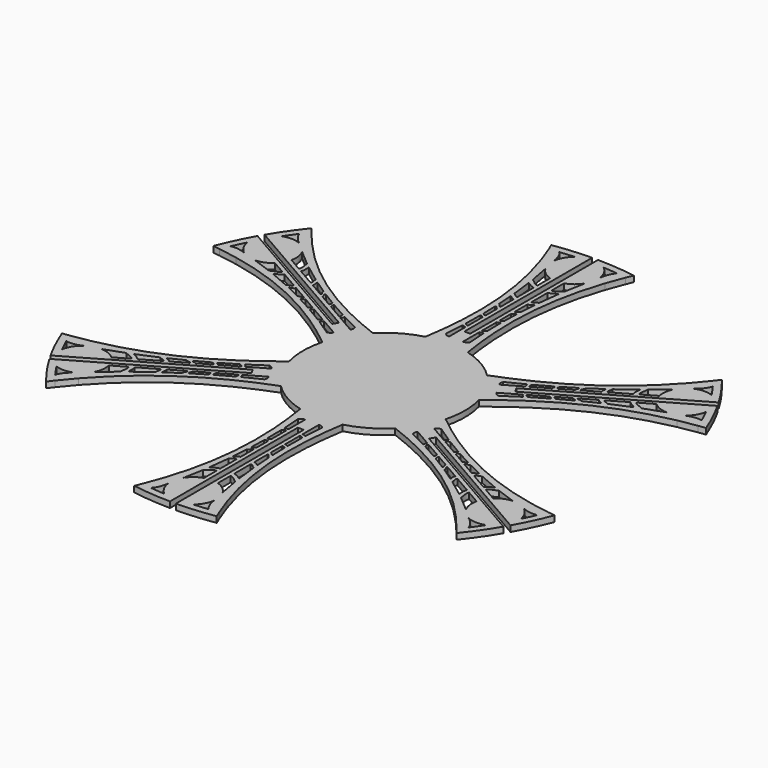
from build123d import *

# Parameters (mm, degrees)
F1_DEPTH = 6.35
F2_COUNT = 6


# Not quite as in the source:
# - a length typed as a fraction of an inch, garbled in the dataset ("3 / 203.2 mm" for 3/8 in), is restored


with BuildPart() as f1:
    # F0 (on Top) → F1 (new body)
    with BuildSketch(Plane.XY):
        with BuildLine():
            ThreePointArc((24.0985074366, 256.3698733068), (24.5345524636, 256.3285113588), (24.9705265041, 256.286407767))
            ThreePointArc((24.9705265041, 256.286407767), (24.9926305398, 256.8930249604), (25, 257.5))
            ThreePointArc((25, 257.5), (24.9791738801, 258.520231477), (24.9167302187, 259.5387631569))
            add(Edge.make_bspline(
                [(24.9167302187, 259.5387631569), (24.6398586668, 258.4897435126), (24.3671164775, 257.4333537767), (24.0985074366, 256.3698733068)],
                knots=[0, 0, 0, 0, 3.5683664228, 3.5683664228, 3.5683664228, 3.5683664228], degree=3))
        make_face()
        with BuildLine():
            ThreePointArc((3.175, 257.4804252269), (8.58681044, 257.3567886932), (13.9948260776, 257.1194174757))
            ThreePointArc((13.9948260776, 257.1194174757), (13.9987064596, 257.3096911541), (14, 257.5))
            ThreePointArc((14, 257.5), (10.9647161386, 266.2048836868), (3.175, 271.1352255207))
            Line((3.175, 271.1352255207), (3.175, 257.4804252269))
        make_face()
        with BuildLine():
            ThreePointArc((3.175, 243.8647744793), (10.845373305, 248.6468718593), (13.9948260776, 257.1194174757))
            ThreePointArc((13.9948260776, 257.1194174757), (8.58681044, 257.3567886932), (3.175, 257.4804252269))
            Line((3.175, 257.4804252269), (3.175, 243.8647744793))
        make_face()
        with BuildLine():
            add(Edge.make_bspline(
                [(34.4843217984, 255.1804881846), (12.7673180552, 190.6958065236), (15.0100402945, 133.2556042085), (22.8586233116, 84.4614310813)],
                knots=[23.4362562465, 23.4362562465, 23.4362562465, 23.4362562465, 198.2251842843, 198.2251842843, 198.2251842843, 198.2251842843], degree=3))
            ThreePointArc((34.4843217984, 255.1804881846), (29.7325665088, 255.7776856741), (24.9705265041, 256.286407767))
            ThreePointArc((24.9705265041, 256.286407767), (23.8907786453, 250.1358506449), (21.3204293609, 244.4447599844))
            add(Edge.make_bspline(
                [(21.3204293609, 244.4447599844), (19.7994681494, 237.3520104746), (18.447355185, 230.0121057952), (17.2650740181, 222.4976243712)],
                knots=[16.6038056007, 16.6038056007, 16.6038056007, 16.6038056007, 39.3732202874, 39.3732202874, 39.3732202874, 39.3732202874], degree=3))
            add(Edge.make_bspline(
                [(17.2650740181, 222.4976243712), (16.9207728297, 220.3092744624), (16.5908746927, 218.106119094), (16.2754038982, 215.8899507729)],
                knots=[39.3732202874, 39.3732202874, 39.3732202874, 39.3732202874, 46.0040765958, 46.0040765958, 46.0040765958, 46.0040765958], degree=3))
            add(Edge.make_bspline(
                [(16.2754038982, 215.8899507729), (15.1982070664, 208.3226908689), (14.2892226929, 200.6037092753), (13.5494178472, 192.8043682385)],
                knots=[46.0040765958, 46.0040765958, 46.0040765958, 46.0040765958, 68.6455937548, 68.6455937548, 68.6455937548, 68.6455937548], degree=3))
            add(Edge.make_bspline(
                [(13.5494178472, 192.8043682385), (13.377969648, 190.9968875439), (13.2156075865, 189.1850909786), (13.0623436996, 187.3698667527)],
                knots=[68.6455937548, 68.6455937548, 68.6455937548, 68.6455937548, 73.8927171936, 73.8927171936, 73.8927171936, 73.8927171936], degree=3))
            add(Edge.make_bspline(
                [(13.0623436996, 187.3698667527), (12.5830867073, 181.6936509129), (12.1927931423, 175.9839188521), (11.891831041, 170.2678288119)],
                knots=[73.8927171936, 73.8927171936, 73.8927171936, 73.8927171936, 90.3005001836, 90.3005001836, 90.3005001836, 90.3005001836], degree=3))
            add(Edge.make_bspline(
                [(11.891831041, 170.2678288119), (11.7934037382, 168.3984262432), (11.7045310241, 166.5283436467), (11.6252257724, 164.6585309992)],
                knots=[90.3005001836, 90.3005001836, 90.3005001836, 90.3005001836, 95.6665373615, 95.6665373615, 95.6665373615, 95.6665373615], degree=3))
            add(Edge.make_bspline(
                [(11.6252257724, 164.6585309992), (11.3941013481, 159.2092150662), (11.244238371, 153.7621919503), (11.1759555056, 148.3409766337)],
                knots=[95.6665373615, 95.6665373615, 95.6665373615, 95.6665373615, 111.3051265697, 111.3051265697, 111.3051265697, 111.3051265697], degree=3))
            add(Edge.make_bspline(
                [(11.1759555056, 148.3409766337), (11.1574760355, 146.8738269174), (11.1449715921, 145.4085673957), (11.1384484917, 143.9456641674)],
                knots=[111.3051265697, 111.3051265697, 111.3051265697, 111.3051265697, 115.5374158962, 115.5374158962, 115.5374158962, 115.5374158962], degree=3))
            add(Edge.make_bspline(
                [(11.1384484917, 143.9456641674), (11.1095814634, 137.471799521), (11.1978516102, 131.0440799553), (11.40380634, 124.7028999515)],
                knots=[115.5374158962, 115.5374158962, 115.5374158962, 115.5374158962, 134.2667943778, 134.2667943778, 134.2667943778, 134.2667943778], degree=3))
            add(Edge.make_bspline(
                [(11.40380634, 124.7028999515), (11.449861348, 123.2849034052), (11.5018011295, 121.8712342374), (11.5596318056, 120.4623441347)],
                knots=[134.2667943778, 134.2667943778, 134.2667943778, 134.2667943778, 138.4550044562, 138.4550044562, 138.4550044562, 138.4550044562], degree=3))
            add(Edge.make_bspline(
                [(11.5596318056, 120.4623441347), (11.848732793, 113.4191700443), (12.2850527804, 106.495429289), (12.869356484, 99.7475520216)],
                knots=[138.4550044562, 138.4550044562, 138.4550044562, 138.4550044562, 159.3922604228, 159.3922604228, 159.3922604228, 159.3922604228], degree=3))
            add(Edge.make_bspline(
                [(12.869356484, 99.7475520216), (13.2640628297, 95.1892547518), (13.7262973279, 90.7112077739), (14.2562957042, 86.3308058157)],
                knots=[159.3922604228, 159.3922604228, 159.3922604228, 159.3922604228, 173.5357062692, 173.5357062692, 173.5357062692, 173.5357062692], degree=3))
            ThreePointArc((14.2562957042, 86.3308058157), (18.5809833933, 85.5043686377), (22.8586233116, 84.4614310813))
        make_face()
        with BuildLine():
            ThreePointArc((24.9705265041, 256.286407767), (29.7325665088, 255.7776856741), (34.4843217984, 255.1804881846))
            add(Edge.make_bspline(
                [(41.5870895219, 274.3661130408), (38.9772182382, 267.9040789576), (36.6154101026, 261.5083662156), (34.4843217984, 255.1804881846)],
                knots=[6.284228985, 6.284228985, 6.284228985, 6.284228985, 23.4362562465, 23.4362562465, 23.4362562465, 23.4362562465], degree=3))
            ThreePointArc((41.5870895219, 274.3661130408), (36.492945437, 275.0900124202), (31.3862552738, 275.719337334))
            add(Edge.make_bspline(
                [(31.3862552738, 275.719337334), (28.0236396939, 273.0873525143), (25.1960325986, 265.6025290489), (24.8841398376, 259.9040766508)],
                knots=[0, 0, 0, 0, 17.0997068871, 17.0997068871, 17.0997068871, 17.0997068871], degree=3))
            ThreePointArc((24.8841398376, 259.9040766508), (24.901104957, 259.7214796696), (24.9167302187, 259.5387631569))
            ThreePointArc((24.9167302187, 259.5387631569), (24.9791738801, 258.520231477), (25, 257.5))
            ThreePointArc((25, 257.5), (24.9926305398, 256.8930249604), (24.9705265041, 256.286407767))
        make_face()
        with BuildLine():
            ThreePointArc((87.5, 0), (69.4851766198, 53.1795094949), (22.8586233116, 84.4614310813))
            ThreePointArc((22.8586233116, 84.4614310813), (18.5809833933, 85.5043686377), (14.2562957042, 86.3308058157))
            ThreePointArc((14.2562957042, 86.3308058157), (10.8863917915, 86.8201386417), (7.5, 87.1779788708))
            ThreePointArc((7.5, 87.1779788708), (5.3391369062, 87.3369544757), (3.175, 87.4423774551))
            ThreePointArc((3.175, 87.4423774551), (0, 87.5), (-3.175, 87.4423774551))
            ThreePointArc((-3.175, 87.4423774551), (-5.3391369062, 87.3369544757), (-7.5, 87.1779788708))
            ThreePointArc((-7.5, 87.1779788708), (-10.8863917915, 86.8201386417), (-14.2562957042, 86.3308058157))
            ThreePointArc((-14.2562957042, 86.3308058157), (-18.5809833933, 85.5043686377), (-22.8586233116, 84.4614310813))
            ThreePointArc((-22.8586233116, 84.4614310813), (-53.1795094949, -69.4851766198), (87.5, 0))
        make_face()
        with BuildLine():
            add(Edge.make_bspline(
                [(-41.5870895219, 274.3661130408), (-38.9772182382, 267.9040789576), (-36.6154101026, 261.5083662156), (-34.4843217984, 255.1804881846)],
                knots=[6.284228985, 6.284228985, 6.284228985, 6.284228985, 23.4362562465, 23.4362562465, 23.4362562465, 23.4362562465], degree=3))
            ThreePointArc((-34.4843217984, 255.1804881846), (-29.7325665088, 255.7776856741), (-24.9705265041, 256.286407767))
            ThreePointArc((-24.9705265041, 256.286407767), (-24.9965807607, 257.9134613325), (-24.9167302187, 259.5387631569))
            ThreePointArc((-24.9167302187, 259.5387631569), (-24.901104957, 259.7214796696), (-24.8841398376, 259.9040766508))
            add(Edge.make_bspline(
                [(-31.3862552738, 275.719337334), (-28.0236396939, 273.0873525143), (-25.1960325986, 265.6025290489), (-24.8841398376, 259.9040766508)],
                knots=[0, 0, 0, 0, 17.0997068871, 17.0997068871, 17.0997068871, 17.0997068871], degree=3))
            ThreePointArc((-31.3862552738, 275.719337334), (-36.492945437, 275.0900124202), (-41.5870895219, 274.3661130408))
        make_face()
        with BuildLine():
            ThreePointArc((-24.9705265041, 256.286407767), (-29.7325665088, 255.7776856741), (-34.4843217984, 255.1804881846))
            add(Edge.make_bspline(
                [(-34.4843217984, 255.1804881846), (-12.7673180552, 190.6958065236), (-15.0100402945, 133.2556042085), (-22.8586233116, 84.4614310813)],
                knots=[23.4362562465, 23.4362562465, 23.4362562465, 23.4362562465, 198.2251842843, 198.2251842843, 198.2251842843, 198.2251842843], degree=3))
            ThreePointArc((-22.8586233116, 84.4614310813), (-18.5809833933, 85.5043686377), (-14.2562957042, 86.3308058157))
            add(Edge.make_bspline(
                [(-12.869356484, 99.7475520216), (-13.2640628297, 95.1892547518), (-13.7262973279, 90.7112077739), (-14.2562957042, 86.3308058157)],
                knots=[159.3922604228, 159.3922604228, 159.3922604228, 159.3922604228, 173.5357062692, 173.5357062692, 173.5357062692, 173.5357062692], degree=3))
            add(Edge.make_bspline(
                [(-11.5596318056, 120.4623441347), (-11.848732793, 113.4191700443), (-12.2850527804, 106.495429289), (-12.869356484, 99.7475520216)],
                knots=[138.4550044562, 138.4550044562, 138.4550044562, 138.4550044562, 159.3922604228, 159.3922604228, 159.3922604228, 159.3922604228], degree=3))
            add(Edge.make_bspline(
                [(-11.40380634, 124.7028999515), (-11.449861348, 123.2849034052), (-11.5018011295, 121.8712342374), (-11.5596318056, 120.4623441347)],
                knots=[134.2667943778, 134.2667943778, 134.2667943778, 134.2667943778, 138.4550044562, 138.4550044562, 138.4550044562, 138.4550044562], degree=3))
            add(Edge.make_bspline(
                [(-11.1384484917, 143.9456641674), (-11.1095814634, 137.471799521), (-11.1978516102, 131.0440799553), (-11.40380634, 124.7028999515)],
                knots=[115.5374158962, 115.5374158962, 115.5374158962, 115.5374158962, 134.2667943778, 134.2667943778, 134.2667943778, 134.2667943778], degree=3))
            add(Edge.make_bspline(
                [(-11.1759555056, 148.3409766337), (-11.1574760355, 146.8738269174), (-11.1449715921, 145.4085673957), (-11.1384484917, 143.9456641674)],
                knots=[111.3051265697, 111.3051265697, 111.3051265697, 111.3051265697, 115.5374158962, 115.5374158962, 115.5374158962, 115.5374158962], degree=3))
            add(Edge.make_bspline(
                [(-11.6252257724, 164.6585309992), (-11.3941013481, 159.2092150662), (-11.244238371, 153.7621919503), (-11.1759555056, 148.3409766337)],
                knots=[95.6665373615, 95.6665373615, 95.6665373615, 95.6665373615, 111.3051265697, 111.3051265697, 111.3051265697, 111.3051265697], degree=3))
            add(Edge.make_bspline(
                [(-11.891831041, 170.2678288119), (-11.7934037382, 168.3984262432), (-11.7045310241, 166.5283436467), (-11.6252257724, 164.6585309992)],
                knots=[90.3005001836, 90.3005001836, 90.3005001836, 90.3005001836, 95.6665373615, 95.6665373615, 95.6665373615, 95.6665373615], degree=3))
            add(Edge.make_bspline(
                [(-13.0623436996, 187.3698667527), (-12.5830867073, 181.6936509129), (-12.1927931423, 175.9839188521), (-11.891831041, 170.2678288119)],
                knots=[73.8927171936, 73.8927171936, 73.8927171936, 73.8927171936, 90.3005001836, 90.3005001836, 90.3005001836, 90.3005001836], degree=3))
            add(Edge.make_bspline(
                [(-13.5494178472, 192.8043682385), (-13.377969648, 190.9968875439), (-13.2156075865, 189.1850909786), (-13.0623436996, 187.3698667527)],
                knots=[68.6455937548, 68.6455937548, 68.6455937548, 68.6455937548, 73.8927171936, 73.8927171936, 73.8927171936, 73.8927171936], degree=3))
            add(Edge.make_bspline(
                [(-16.2754038982, 215.8899507729), (-15.1982070664, 208.3226908689), (-14.2892226929, 200.6037092753), (-13.5494178472, 192.8043682385)],
                knots=[46.0040765958, 46.0040765958, 46.0040765958, 46.0040765958, 68.6455937548, 68.6455937548, 68.6455937548, 68.6455937548], degree=3))
            add(Edge.make_bspline(
                [(-17.2650740181, 222.4976243712), (-16.9207728297, 220.3092744624), (-16.5908746927, 218.106119094), (-16.2754038982, 215.8899507729)],
                knots=[39.3732202874, 39.3732202874, 39.3732202874, 39.3732202874, 46.0040765958, 46.0040765958, 46.0040765958, 46.0040765958], degree=3))
            add(Edge.make_bspline(
                [(-21.3204293609, 244.4447599844), (-19.7994681494, 237.3520104746), (-18.447355185, 230.0121057952), (-17.2650740181, 222.4976243712)],
                knots=[16.6038056007, 16.6038056007, 16.6038056007, 16.6038056007, 39.3732202874, 39.3732202874, 39.3732202874, 39.3732202874], degree=3))
            ThreePointArc((-21.3204293609, 244.4447599844), (-23.8907786453, 250.1358506449), (-24.9705265041, 256.286407767))
        make_face()
        with BuildLine():
            add(Edge.make_bspline(
                [(-17.2650740181, 222.4976243712), (-13.0134568191, 219.9089487239), (-11.2873415643, 216.6422307491), (-7.5, 216.5923267603)],
                knots=[0, 0, 0, 0, 11.4118013675, 11.4118013675, 11.4118013675, 11.4118013675], degree=3))
            add(Edge.make_bspline(
                [(-17.2650740181, 222.4976243712), (-16.9207728297, 220.3092744624), (-16.5908746927, 218.106119094), (-16.2754038982, 215.8899507729)],
                knots=[39.3732202874, 39.3732202874, 39.3732202874, 39.3732202874, 46.0040765958, 46.0040765958, 46.0040765958, 46.0040765958], degree=3))
            add(Edge.make_bspline(
                [(-16.2754038982, 215.8899507729), (-12.5103608703, 213.8302643566), (-11.8700430909, 212.4467641115), (-7.5, 211.5250229836)],
                knots=[0, 0, 0, 0, 9.801036077, 9.801036077, 9.801036077, 9.801036077], degree=3))
            Line((-7.5, 211.5250229836), (-7.5, 216.5923267603))
        make_face()
        with BuildLine():
            add(Edge.make_bspline(
                [(-13.5494178472, 192.8043682385), (-10.0457689154, 191.3002797398), (-10.2384781645, 189.022153616), (-7.5, 189.5666867495)],
                knots=[0, 0, 0, 0, 6.8613437252, 6.8613437252, 6.8613437252, 6.8613437252], degree=3))
            add(Edge.make_bspline(
                [(-13.5494178472, 192.8043682385), (-13.377969648, 190.9968875439), (-13.2156075865, 189.1850909786), (-13.0623436996, 187.3698667527)],
                knots=[68.6455937548, 68.6455937548, 68.6455937548, 68.6455937548, 73.8927171936, 73.8927171936, 73.8927171936, 73.8927171936], degree=3))
            add(Edge.make_bspline(
                [(-13.0623436996, 187.3698667527), (-10.2409727406, 186.262742786), (-10.2384781645, 184.243991971), (-7.5, 184.4993829727)],
                knots=[0, 0, 0, 0, 6.2593405854, 6.2593405854, 6.2593405854, 6.2593405854], degree=3))
            Line((-7.5, 184.4993829727), (-7.5, 189.5666867495))
        make_face()
        with BuildLine():
            add(Edge.make_bspline(
                [(-11.891831041, 170.2678288119), (-9.259641322, 169.3483605489), (-9.8297276348, 166.1768704653), (-7.5, 166.491702199)],
                knots=[0, 0, 0, 0, 5.7920041513, 5.7920041513, 5.7920041513, 5.7920041513], degree=3))
            add(Edge.make_bspline(
                [(-11.891831041, 170.2678288119), (-11.7934037382, 168.3984262432), (-11.7045310241, 166.5283436467), (-11.6252257724, 164.6585309992)],
                knots=[90.3005001836, 90.3005001836, 90.3005001836, 90.3005001836, 95.6665373615, 95.6665373615, 95.6665373615, 95.6665373615], degree=3))
            add(Edge.make_bspline(
                [(-11.6252257724, 164.6585309992), (-8.90752234, 165.1033413686), (-9.8926938884, 162.4619066715), (-7.5, 162.2730046511)],
                knots=[0, 0, 0, 0, 4.7653146413, 4.7653146413, 4.7653146413, 4.7653146413], degree=3))
            Line((-7.5, 162.2730046511), (-7.5, 166.491702199))
        make_face()
        with BuildLine():
            add(Edge.make_bspline(
                [(-11.1759555056, 148.3409766337), (-11.1574760355, 146.8738269174), (-11.1449715921, 145.4085673957), (-11.1384484917, 143.9456641674)],
                knots=[111.3051265697, 111.3051265697, 111.3051265697, 111.3051265697, 115.5374158962, 115.5374158962, 115.5374158962, 115.5374158962], degree=3))
            add(Edge.make_bspline(
                [(-11.1384484917, 143.9456641674), (-8.4912590683, 144.0353989601), (-9.1877372184, 142.4406170845), (-7.5, 142.7544057369)],
                knots=[0, 0, 0, 0, 3.8284989323, 3.8284989323, 3.8284989323, 3.8284989323], degree=3))
            Line((-7.5, 142.7544057369), (-7.5, 146.8565165997))
            add(Edge.make_bspline(
                [(-11.1759555056, 148.3409766337), (-9.7026852891, 146.906927228), (-9.2796140531, 146.3913172483), (-7.5, 146.8565165997)],
                knots=[0, 0, 0, 0, 3.9643751679, 3.9643751679, 3.9643751679, 3.9643751679], degree=3))
        make_face()
        with BuildLine():
            add(Edge.make_bspline(
                [(-11.40380634, 124.7028999515), (-11.449861348, 123.2849034052), (-11.5018011295, 121.8712342374), (-11.5596318056, 120.4623441347)],
                knots=[134.2667943778, 134.2667943778, 134.2667943778, 134.2667943778, 138.4550044562, 138.4550044562, 138.4550044562, 138.4550044562], degree=3))
            add(Edge.make_bspline(
                [(-11.5596318056, 120.4623441347), (-9.5880907525, 119.8675970578), (-9.5183962158, 119.5819102936), (-7.5, 119.7053417563)],
                knots=[0, 0, 0, 0, 4.1296080926, 4.1296080926, 4.1296080926, 4.1296080926], degree=3))
            Line((-7.5, 119.7053417563), (-7.5, 122.7562793089))
            add(Edge.make_bspline(
                [(-11.40380634, 124.7028999515), (-9.5969793375, 123.429948461), (-9.4491818808, 122.6324219398), (-7.5, 122.7562793089)],
                knots=[0, 0, 0, 0, 4.3622283143, 4.3622283143, 4.3622283143, 4.3622283143], degree=3))
        make_face()
        with BuildLine():
            add(Edge.make_bspline(
                [(-12.869356484, 99.7475520216), (-13.2640628297, 95.1892547518), (-13.7262973279, 90.7112077739), (-14.2562957042, 86.3308058157)],
                knots=[159.3922604228, 159.3922604228, 159.3922604228, 159.3922604228, 173.5357062692, 173.5357062692, 173.5357062692, 173.5357062692], degree=3))
            ThreePointArc((-14.2562957042, 86.3308058157), (-10.8863917915, 86.8201386417), (-7.5, 87.1779788708))
            Line((-7.5, 87.1779788708), (-7.5, 97.2476452589))
            add(Edge.make_bspline(
                [(-12.869356484, 99.7475520216), (-10.8381348679, 97.5883237043), (-10.0787932936, 97.1908478477), (-7.5, 97.2476452589)],
                knots=[0, 0, 0, 0, 5.9227968794, 5.9227968794, 5.9227968794, 5.9227968794], degree=3))
        make_face()
        with BuildLine():
            ThreePointArc((21.3204293609, 244.4447599844), (23.8907786453, 250.1358506449), (24.9705265041, 256.286407767))
            ThreePointArc((24.9705265041, 256.286407767), (24.5345524636, 256.3285113588), (24.0985074366, 256.3698733068))
            add(Edge.make_bspline(
                [(24.0985074366, 256.3698733068), (23.1172638083, 252.4849205467), (22.1911762658, 248.5053432761), (21.3204293609, 244.4447599844)],
                knots=[3.5683664228, 3.5683664228, 3.5683664228, 3.5683664228, 16.6038056007, 16.6038056007, 16.6038056007, 16.6038056007], degree=3))
        make_face()
        with BuildLine():
            ThreePointArc((-24.0985074366, 256.3698733068), (-24.5345524636, 256.3285113588), (-24.9705265041, 256.286407767))
            ThreePointArc((-24.9705265041, 256.286407767), (-23.8907786453, 250.1358506449), (-21.3204293609, 244.4447599844))
            add(Edge.make_bspline(
                [(-24.0985074366, 256.3698733068), (-23.1172638083, 252.4849205467), (-22.1911762658, 248.5053432761), (-21.3204293609, 244.4447599844)],
                knots=[3.5683664228, 3.5683664228, 3.5683664228, 3.5683664228, 16.6038056007, 16.6038056007, 16.6038056007, 16.6038056007], degree=3))
        make_face()
        with BuildLine():
            ThreePointArc((-24.9167302187, 259.5387631569), (-24.9965807607, 257.9134613325), (-24.9705265041, 256.286407767))
            ThreePointArc((-24.9705265041, 256.286407767), (-24.5345524636, 256.3285113588), (-24.0985074366, 256.3698733068))
            add(Edge.make_bspline(
                [(-24.9167302187, 259.5387631569), (-24.6398586668, 258.4897435126), (-24.3671164775, 257.4333537767), (-24.0985074366, 256.3698733068)],
                knots=[0, 0, 0, 0, 3.5683664228, 3.5683664228, 3.5683664228, 3.5683664228], degree=3))
        make_face()
        with BuildLine():
            add(Edge.make_bspline(
                [(24.0985074366, 256.3698733068), (23.1172638083, 252.4849205467), (22.1911762658, 248.5053432761), (21.3204293609, 244.4447599844)],
                knots=[3.5683664228, 3.5683664228, 3.5683664228, 3.5683664228, 16.6038056007, 16.6038056007, 16.6038056007, 16.6038056007], degree=3))
            ThreePointArc((24.0985074366, 256.3698733068), (19.0503535051, 256.794341899), (13.9948260776, 257.1194174757))
            ThreePointArc((13.9948260776, 257.1194174757), (10.845373305, 248.6468718593), (3.175, 243.8647744793))
            Line((3.175, 243.8647744793), (3.175, 232.7024320749))
            ThreePointArc((3.175, 232.7024320749), (5.358553742, 233.0810339737), (7.5, 233.6515199646))
            ThreePointArc((7.5, 233.6515199646), (15.3875857323, 237.7966448204), (21.3204293609, 244.4447599844))
        make_face()
        with BuildLine():
            ThreePointArc((31.3862552738, 275.719337334), (36.492945437, 275.0900124202), (41.5870895219, 274.3661130408))
            add(Edge.make_bspline(
                [(44.5564859897, 281.4955053926), (43.532819192, 279.1101881008), (42.543304698, 276.7336991732), (41.5870895219, 274.3661130408)],
                knots=[0, 0, 0, 0, 6.284228985, 6.284228985, 6.284228985, 6.284228985], degree=3))
            ThreePointArc((44.5564859897, 281.4955053926), (23.9293365456, 283.9936387536), (3.175, 284.9823141442))
            Line((3.175, 284.9823141442), (3.175, 282.2975679251))
            ThreePointArc((3.175, 282.2975679251), (9.7289002268, 280.5292965672), (15.5655019991, 277.0631067961))
            ThreePointArc((15.5655019991, 277.0631067961), (23.4854914116, 276.5043972402), (31.3862552738, 275.719337334))
        make_face()
        with BuildLine():
            ThreePointArc((13.9948260776, 257.1194174757), (19.0503535051, 256.794341899), (24.0985074366, 256.3698733068))
            add(Edge.make_bspline(
                [(24.9167302187, 259.5387631569), (24.6398586668, 258.4897435126), (24.3671164775, 257.4333537767), (24.0985074366, 256.3698733068)],
                knots=[0, 0, 0, 0, 3.5683664228, 3.5683664228, 3.5683664228, 3.5683664228], degree=3))
            ThreePointArc((24.9167302187, 259.5387631569), (24.901104957, 259.7214796696), (24.8841398376, 259.9040766508))
            ThreePointArc((24.8841398376, 259.9040766508), (21.9693299866, 269.4309907358), (15.5655019991, 277.0631067961))
            ThreePointArc((15.5655019991, 277.0631067961), (9.3725896824, 277.3416747671), (3.175, 277.4818361172))
            Line((3.175, 277.4818361172), (3.175, 271.1352255207))
            ThreePointArc((3.175, 271.1352255207), (10.9647161386, 266.2048836868), (14, 257.5))
            ThreePointArc((14, 257.5), (13.9987064596, 257.3096911541), (13.9948260776, 257.1194174757))
        make_face()
        with BuildLine():
            ThreePointArc((3.175, 277.4818361172), (9.3725896824, 277.3416747671), (15.5655019991, 277.0631067961))
            ThreePointArc((15.5655019991, 277.0631067961), (9.7289002268, 280.5292965672), (3.175, 282.2975679251))
            Line((3.175, 282.2975679251), (3.175, 277.4818361172))
        make_face()
        with BuildLine():
            ThreePointArc((-3.175, 232.7024320749), (-5.358553742, 233.0810339737), (-7.5, 233.6515199646))
            Line((-7.5, 233.6515199646), (-7.5, 216.5923267603))
            Line((-7.5, 216.5923267603), (-7.5, 211.5250229836))
            Line((-7.5, 211.5250229836), (-7.5, 189.5666867495))
            Line((-7.5, 189.5666867495), (-7.5, 184.4993829727))
            Line((-7.5, 184.4993829727), (-7.5, 166.491702199))
            Line((-7.5, 166.491702199), (-7.5, 162.2730046511))
            Line((-7.5, 162.2730046511), (-7.5, 146.8565165997))
            Line((-7.5, 146.8565165997), (-7.5, 142.7544057369))
            Line((-7.5, 142.7544057369), (-7.5, 122.7562793089))
            Line((-7.5, 122.7562793089), (-7.5, 119.7053417563))
            Line((-7.5, 119.7053417563), (-7.5, 97.2476452589))
            Line((-7.5, 97.2476452589), (-7.5, 87.1779788708))
            ThreePointArc((-7.5, 87.1779788708), (-5.3391369062, 87.3369544757), (-3.175, 87.4423774551))
            Line((-3.175, 87.4423774551), (-3.175, 112.4423774551))
            Line((-3.175, 112.4423774551), (-3.175, 232.7024320749))
        make_face()
        with BuildLine():
            add(Edge.make_bspline(
                [(17.2650740181, 222.4976243712), (16.9207728297, 220.3092744624), (16.5908746927, 218.106119094), (16.2754038982, 215.8899507729)],
                knots=[39.3732202874, 39.3732202874, 39.3732202874, 39.3732202874, 46.0040765958, 46.0040765958, 46.0040765958, 46.0040765958], degree=3))
            add(Edge.make_bspline(
                [(17.2650740181, 222.4976243712), (13.0134568191, 219.9089487239), (11.2873415643, 216.6422307491), (7.5, 216.5923267603)],
                knots=[0, 0, 0, 0, 11.4118013675, 11.4118013675, 11.4118013675, 11.4118013675], degree=3))
            Line((7.5, 216.5923267603), (7.5, 211.5250229836))
            add(Edge.make_bspline(
                [(16.2754038982, 215.8899507729), (12.5103608703, 213.8302643566), (11.8700430909, 212.4467641115), (7.5, 211.5250229836)],
                knots=[0, 0, 0, 0, 9.801036077, 9.801036077, 9.801036077, 9.801036077], degree=3))
        make_face()
        with BuildLine():
            add(Edge.make_bspline(
                [(13.5494178472, 192.8043682385), (13.377969648, 190.9968875439), (13.2156075865, 189.1850909786), (13.0623436996, 187.3698667527)],
                knots=[68.6455937548, 68.6455937548, 68.6455937548, 68.6455937548, 73.8927171936, 73.8927171936, 73.8927171936, 73.8927171936], degree=3))
            add(Edge.make_bspline(
                [(13.5494178472, 192.8043682385), (10.0457689154, 191.3002797398), (10.2384781645, 189.022153616), (7.5, 189.5666867495)],
                knots=[0, 0, 0, 0, 6.8613437252, 6.8613437252, 6.8613437252, 6.8613437252], degree=3))
            Line((7.5, 189.5666867495), (7.5, 184.4993829727))
            add(Edge.make_bspline(
                [(13.0623436996, 187.3698667527), (10.2409727406, 186.262742786), (10.2384781645, 184.243991971), (7.5, 184.4993829727)],
                knots=[0, 0, 0, 0, 6.2593405854, 6.2593405854, 6.2593405854, 6.2593405854], degree=3))
        make_face()
        with BuildLine():
            add(Edge.make_bspline(
                [(11.891831041, 170.2678288119), (11.7934037382, 168.3984262432), (11.7045310241, 166.5283436467), (11.6252257724, 164.6585309992)],
                knots=[90.3005001836, 90.3005001836, 90.3005001836, 90.3005001836, 95.6665373615, 95.6665373615, 95.6665373615, 95.6665373615], degree=3))
            add(Edge.make_bspline(
                [(11.891831041, 170.2678288119), (9.259641322, 169.3483605489), (9.8297276348, 166.1768704653), (7.5, 166.491702199)],
                knots=[0, 0, 0, 0, 5.7920041513, 5.7920041513, 5.7920041513, 5.7920041513], degree=3))
            Line((7.5, 166.491702199), (7.5, 162.2730046511))
            add(Edge.make_bspline(
                [(11.6252257724, 164.6585309992), (8.90752234, 165.1033413686), (9.8926938884, 162.4619066715), (7.5, 162.2730046511)],
                knots=[0, 0, 0, 0, 4.7653146413, 4.7653146413, 4.7653146413, 4.7653146413], degree=3))
        make_face()
        with BuildLine():
            add(Edge.make_bspline(
                [(11.1384484917, 143.9456641674), (8.4912590683, 144.0353989601), (9.1877372184, 142.4406170845), (7.5, 142.7544057369)],
                knots=[0, 0, 0, 0, 3.8284989323, 3.8284989323, 3.8284989323, 3.8284989323], degree=3))
            add(Edge.make_bspline(
                [(11.1759555056, 148.3409766337), (11.1574760355, 146.8738269174), (11.1449715921, 145.4085673957), (11.1384484917, 143.9456641674)],
                knots=[111.3051265697, 111.3051265697, 111.3051265697, 111.3051265697, 115.5374158962, 115.5374158962, 115.5374158962, 115.5374158962], degree=3))
            add(Edge.make_bspline(
                [(11.1759555056, 148.3409766337), (9.7026852891, 146.906927228), (9.2796140531, 146.3913172483), (7.5, 146.8565165997)],
                knots=[0, 0, 0, 0, 3.9643751679, 3.9643751679, 3.9643751679, 3.9643751679], degree=3))
            Line((7.5, 146.8565165997), (7.5, 142.7544057369))
        make_face()
        with BuildLine():
            add(Edge.make_bspline(
                [(11.5596318056, 120.4623441347), (9.5880907525, 119.8675970578), (9.5183962158, 119.5819102936), (7.5, 119.7053417563)],
                knots=[0, 0, 0, 0, 4.1296080926, 4.1296080926, 4.1296080926, 4.1296080926], degree=3))
            add(Edge.make_bspline(
                [(11.40380634, 124.7028999515), (11.449861348, 123.2849034052), (11.5018011295, 121.8712342374), (11.5596318056, 120.4623441347)],
                knots=[134.2667943778, 134.2667943778, 134.2667943778, 134.2667943778, 138.4550044562, 138.4550044562, 138.4550044562, 138.4550044562], degree=3))
            add(Edge.make_bspline(
                [(11.40380634, 124.7028999515), (9.5969793375, 123.429948461), (9.4491818808, 122.6324219398), (7.5, 122.7562793089)],
                knots=[0, 0, 0, 0, 4.3622283143, 4.3622283143, 4.3622283143, 4.3622283143], degree=3))
            Line((7.5, 122.7562793089), (7.5, 119.7053417563))
        make_face()
        with BuildLine():
            ThreePointArc((7.5, 87.1779788708), (10.8863917915, 86.8201386417), (14.2562957042, 86.3308058157))
            add(Edge.make_bspline(
                [(12.869356484, 99.7475520216), (13.2640628297, 95.1892547518), (13.7262973279, 90.7112077739), (14.2562957042, 86.3308058157)],
                knots=[159.3922604228, 159.3922604228, 159.3922604228, 159.3922604228, 173.5357062692, 173.5357062692, 173.5357062692, 173.5357062692], degree=3))
            add(Edge.make_bspline(
                [(12.869356484, 99.7475520216), (10.8381348679, 97.5883237043), (10.0787932936, 97.1908478477), (7.5, 97.2476452589)],
                knots=[0, 0, 0, 0, 5.9227968794, 5.9227968794, 5.9227968794, 5.9227968794], degree=3))
            Line((7.5, 97.2476452589), (7.5, 87.1779788708))
        make_face()
        with BuildLine():
            Line((7.5, 216.5923267603), (7.5, 233.6515199646))
            ThreePointArc((7.5, 233.6515199646), (5.358553742, 233.0810339737), (3.175, 232.7024320749))
            Line((3.175, 232.7024320749), (3.175, 112.4423774551))
            Line((3.175, 112.4423774551), (3.175, 87.4423774551))
            ThreePointArc((3.175, 87.4423774551), (5.3391369062, 87.3369544757), (7.5, 87.1779788708))
            Line((7.5, 87.1779788708), (7.5, 97.2476452589))
            Line((7.5, 97.2476452589), (7.5, 119.7053417563))
            Line((7.5, 119.7053417563), (7.5, 122.7562793089))
            Line((7.5, 122.7562793089), (7.5, 142.7544057369))
            Line((7.5, 142.7544057369), (7.5, 146.8565165997))
            Line((7.5, 146.8565165997), (7.5, 162.2730046511))
            Line((7.5, 162.2730046511), (7.5, 166.491702199))
            Line((7.5, 166.491702199), (7.5, 184.4993829727))
            Line((7.5, 184.4993829727), (7.5, 189.5666867495))
            Line((7.5, 189.5666867495), (7.5, 211.5250229836))
            Line((7.5, 211.5250229836), (7.5, 216.5923267603))
        make_face()
        with BuildLine():
            ThreePointArc((-13.9948260776, 257.1194174757), (-19.0503535051, 256.794341899), (-24.0985074366, 256.3698733068))
            add(Edge.make_bspline(
                [(-24.0985074366, 256.3698733068), (-23.1172638083, 252.4849205467), (-22.1911762658, 248.5053432761), (-21.3204293609, 244.4447599844)],
                knots=[3.5683664228, 3.5683664228, 3.5683664228, 3.5683664228, 16.6038056007, 16.6038056007, 16.6038056007, 16.6038056007], degree=3))
            ThreePointArc((-21.3204293609, 244.4447599844), (-15.3875857323, 237.7966448204), (-7.5, 233.6515199646))
            ThreePointArc((-7.5, 233.6515199646), (-5.358553742, 233.0810339737), (-3.175, 232.7024320749))
            Line((-3.175, 232.7024320749), (-3.175, 243.8647744793))
            ThreePointArc((-3.175, 243.8647744793), (-10.845373305, 248.6468718593), (-13.9948260776, 257.1194174757))
        make_face()
        with BuildLine():
            ThreePointArc((-3.175, 257.4804252269), (-8.58681044, 257.3567886932), (-13.9948260776, 257.1194174757))
            ThreePointArc((-13.9948260776, 257.1194174757), (-10.845373305, 248.6468718593), (-3.175, 243.8647744793))
            Line((-3.175, 243.8647744793), (-3.175, 257.4804252269))
        make_face()
        with BuildLine():
            ThreePointArc((-3.175, 271.1352255207), (-11.0820327861, 266.0550306445), (-13.9948260776, 257.1194174757))
            ThreePointArc((-13.9948260776, 257.1194174757), (-8.58681044, 257.3567886932), (-3.175, 257.4804252269))
            Line((-3.175, 257.4804252269), (-3.175, 271.1352255207))
        make_face()
        with BuildLine():
            add(Edge.make_bspline(
                [(-24.9167302187, 259.5387631569), (-24.6398586668, 258.4897435126), (-24.3671164775, 257.4333537767), (-24.0985074366, 256.3698733068)],
                knots=[0, 0, 0, 0, 3.5683664228, 3.5683664228, 3.5683664228, 3.5683664228], degree=3))
            ThreePointArc((-24.0985074366, 256.3698733068), (-19.0503535051, 256.794341899), (-13.9948260776, 257.1194174757))
            ThreePointArc((-13.9948260776, 257.1194174757), (-11.0820327861, 266.0550306445), (-3.175, 271.1352255207))
            Line((-3.175, 271.1352255207), (-3.175, 277.4818361172))
            ThreePointArc((-3.175, 277.4818361172), (-9.3725896824, 277.3416747671), (-15.5655019991, 277.0631067961))
            ThreePointArc((-15.5655019991, 277.0631067961), (-21.9693299866, 269.4309907358), (-24.8841398376, 259.9040766508))
            ThreePointArc((-24.8841398376, 259.9040766508), (-24.901104957, 259.7214796696), (-24.9167302187, 259.5387631569))
        make_face()
        with BuildLine():
            ThreePointArc((-3.175, 282.2975679251), (-9.7289002268, 280.5292965672), (-15.5655019991, 277.0631067961))
            ThreePointArc((-15.5655019991, 277.0631067961), (-9.3725896824, 277.3416747671), (-3.175, 277.4818361172))
            Line((-3.175, 277.4818361172), (-3.175, 282.2975679251))
        make_face()
        with BuildLine():
            add(Edge.make_bspline(
                [(-44.5564859897, 281.4955053926), (-43.532819192, 279.1101881008), (-42.543304698, 276.7336991732), (-41.5870895219, 274.3661130408)],
                knots=[0, 0, 0, 0, 6.284228985, 6.284228985, 6.284228985, 6.284228985], degree=3))
            ThreePointArc((-41.5870895219, 274.3661130408), (-36.492945437, 275.0900124202), (-31.3862552738, 275.719337334))
            ThreePointArc((-31.3862552738, 275.719337334), (-23.4854914116, 276.5043972402), (-15.5655019991, 277.0631067961))
            ThreePointArc((-15.5655019991, 277.0631067961), (-9.7289002268, 280.5292965672), (-3.175, 282.2975679251))
            Line((-3.175, 282.2975679251), (-3.175, 284.9823141442))
            ThreePointArc((-3.175, 284.9823141442), (-23.9293365456, 283.9936387536), (-44.5564859897, 281.4955053926))
        make_face()
        with BuildLine():
            ThreePointArc((-3.175, 87.4423774551), (0, 87.5), (3.175, 87.4423774551))
            Line((3.175, 87.4423774551), (3.175, 112.4423774551))
            Line((3.175, 112.4423774551), (-3.175, 112.4423774551))
            Line((-3.175, 112.4423774551), (-3.175, 87.4423774551))
        make_face()
    extrude(amount=-F1_DEPTH)

    # F2: F1 ×6 about axis
    f2_axis = Axis((0, 0, 0), (0, 0, 1))


with BuildPart() as f1_1:
    add(f1.part)
    for i in range(1, F2_COUNT):
        add(f1.part.rotate(f2_axis, i * 360 / F2_COUNT))


solid = f1_1.part
